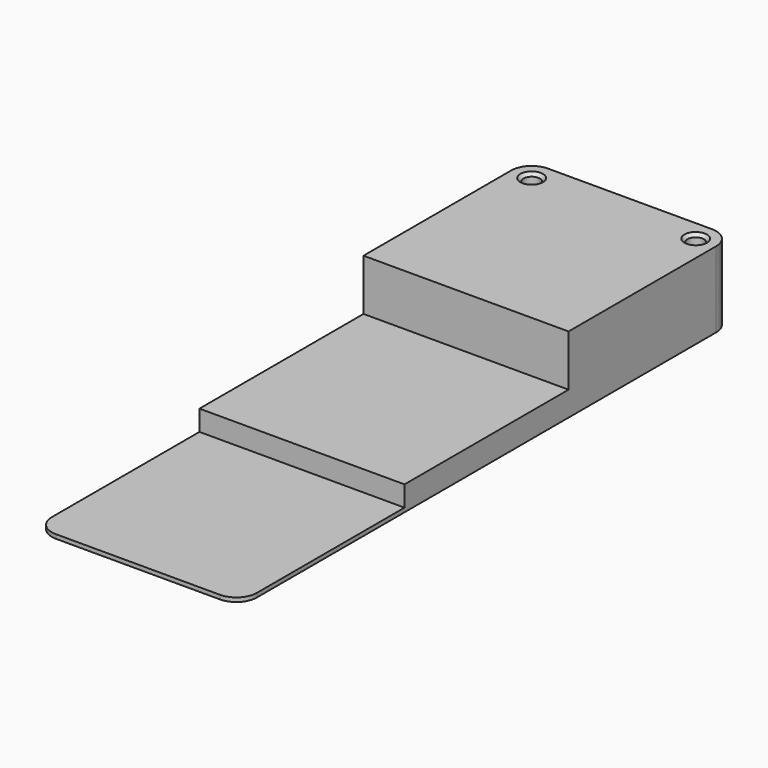
from build123d import *

# Parameters (mm, degrees)
F0_W     = 100
F0_H     = 300
F1_DEPTH = 2
F2_W     = 100
F2_H     = 200
F3_DEPTH = 10
F4_W     = 100
F4_H     = 100
F5_DEPTH = 25
F6_R     = 10
F7_R     = 4
F8_DEPTH = 37.001
F9_SIZE  = 1.5


# Not quite as in the source:
# - a pattern or mirror of a feature is missing from the dataset's text; its kind, count and spacing are read off the source's solid


with BuildPart() as f1:
    # F0 (on Top) → F1 (new body)
    with BuildSketch(Plane.XY):
        Rectangle(F0_W, F0_H)
    extrude(amount=F1_DEPTH)

    # F2 (on face) → F3 (join)
    with BuildSketch(Plane.XY.offset(2)):
        with Locations((0, 50)):
            Rectangle(F2_W, F2_H)
    extrude(amount=F3_DEPTH)

    # F4 (on face) → F5 (join)
    with BuildSketch(Plane.XY.offset(12)):
        with Locations((0, 100)):
            Rectangle(F4_W, F4_H)
    extrude(amount=F5_DEPTH)

    # F6
    f6_edges = [f1.edges().sort_by_distance(p)[0] for p in [
        (-50, 150, 18.5),
        (-50, -150, 1),
        (50, -150, 1),
        (50, 150, 18.5),
    ]]
    fillet(f6_edges, radius=F6_R)

    # F7 (on face) → F8 (cut, through all)
    with BuildSketch(Plane.XY.offset(37)):
        with Locations((-40, 140)):
            Circle(F7_R)
    f8 = extrude(amount=-F8_DEPTH, mode=Mode.SUBTRACT)

    # F8_copies: F8 across plane
    add(f8.mirror(Plane(origin=(0, 0, 0), x_dir=(0, 0, 1), z_dir=(1, 0, 0))), mode=Mode.SUBTRACT)

    # F9
    f9_edges = [f1.edges().sort_by_distance(p)[0] for p in [
        (-44, 140, 37),
        (-36, 140, 18.5),
        (-44, 140, 0),
        (44, 140, 0),
        (44, 140, 37),
    ]]
    chamfer(f9_edges, length=F9_SIZE)


solid = f1.part
